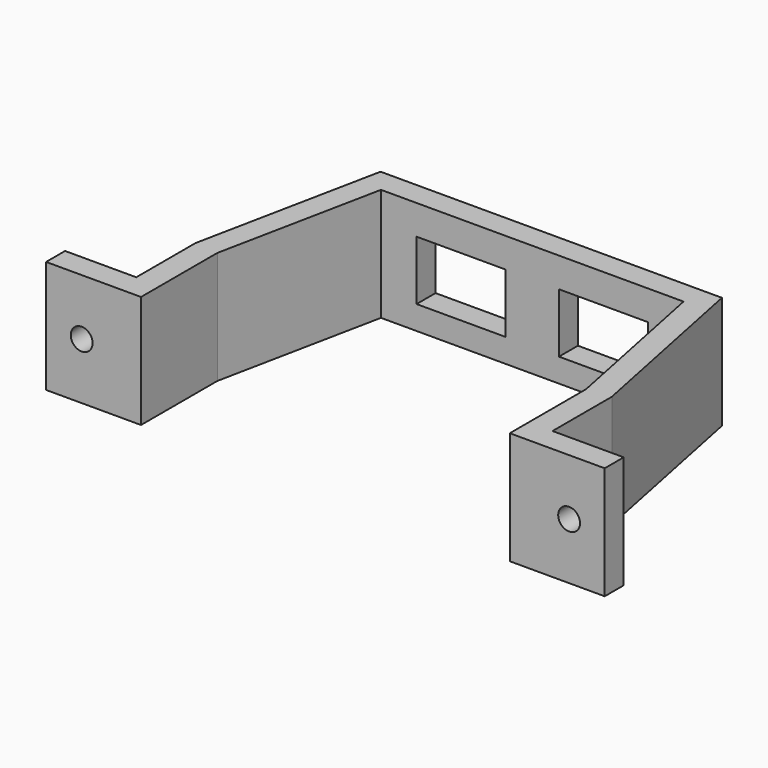
from build123d import *

# Parameters (mm, degrees)
F1_DEPTH = 30.1625
F2_W     = 23.8125
F2_H     = 15.875
F3_DEPTH = 6.35
F4_R     = 2.921
F5_DEPTH = 6.35


# Not quite as in the source:
# - a feature names something its author has since deleted; it is built from what else it names


with BuildPart() as f1:
    # F0 (on Top) → F1 (new body)
    with BuildSketch(Plane.XY):
        Polygon((-40.48125, 0), (0, 0), (40.48125, 0), (49.3395, -43.65625), (49.3395, -69.1896), (55.6895, -69.1896), (74.7395, -69.1896), (74.7395, -62.8396), (55.6895, -62.8396), (55.6895, -43.0185116827), (45.6721801749, 6.35), (0, 6.35), (-45.6721801749, 6.35), (-55.6895, -43.0185116827), (-55.6895, -62.8396), (-74.7395, -62.8396), (-74.7395, -69.1896), (-55.6895, -69.1896), (-49.3395, -69.1896), (-49.3395, -43.65625), align=None)
    extrude(amount=F1_DEPTH)

    # F2 (on face) → F3 (cut, through all)
    with BuildSketch(Plane.XZ):
        with Locations((-19.05, 14.2875)):
            Rectangle(F2_W, F2_H)
        with Locations((19.05, 14.2875)):
            Rectangle(F2_W, F2_H)
    extrude(amount=-F3_DEPTH, mode=Mode.SUBTRACT)

    # F4 (on face) → F5 (cut, through all)
    with BuildSketch(Plane(origin=(0, -62.8396, 0), x_dir=(-1, 0, 0), z_dir=(0, 1, 0))):
        with Locations((65.2145, 15.08125)):
            Circle(F4_R)
        with Locations((-65.2145, 15.08125)):
            Circle(F4_R)
    extrude(amount=-F5_DEPTH, mode=Mode.SUBTRACT)


solid = f1.part
